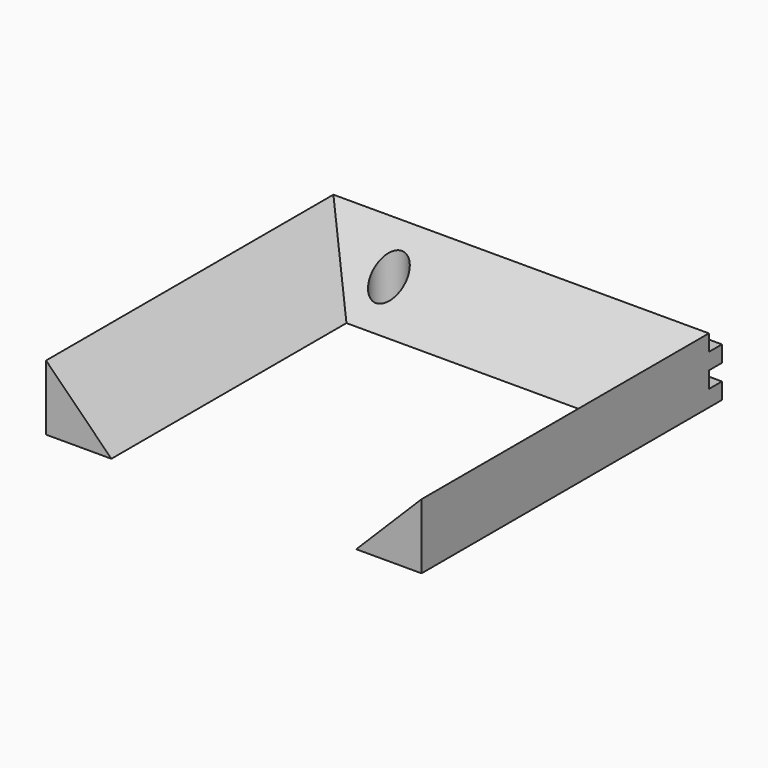
from build123d import *

# Parameters (mm, degrees)
F0_W     = 50.8
F0_H     = 228.6
F1_DEPTH = 50.8
F2_SIZE  = 50.79999
F4_R     = 12.7
F5_DEPTH = 63.5
F3_W     = 292.1
F3_H     = 12.7
F6_DEPTH = 12.7


# Not quite as in the source:
# - a fillet or chamfer is up to 0.001 mm smaller than in the source, because OpenCascade refuses the exact size


with BuildPart() as f1:
    # F0 (on Top) → F1 (new body)
    with BuildSketch(Plane.XY):
        with Locations((25.4, -114.3)):
            Rectangle(F0_W, F0_H)
        Polygon((0, 50.8), (0, 0), (50.8, 0), (241.3, 0), (292.1, 0), (292.1, 50.8), align=None)
        with Locations((266.7, -114.3)):
            Rectangle(F0_W, F0_H)
    extrude(amount=F1_DEPTH)

    # F2 (size 50.8 in the source; OpenCascade refuses exactly that, so slightly less here)
    f2_edges = [f1.edges().sort_by_distance(p)[0] for p in [
        (50.8, -114.3, 50.8),
        (146.05, 0, 50.8),
        (241.3, -114.3, 50.8),
    ]]
    chamfer(f2_edges, length=F2_SIZE)

    # F4 (on face) → F5 (cut)
    with BuildSketch(Plane(origin=(0, 0, 0), x_dir=(1, 0, 0), z_dir=(0, 0, -1))):
        with Locations((63.5, -25.4)):
            Circle(F4_R)
    extrude(amount=-F5_DEPTH, mode=Mode.SUBTRACT)

    # F3 (on face) → F6 (join)
    with BuildSketch(Plane(origin=(0, 50.8, 0), x_dir=(-1, 0, 0), z_dir=(0, 1, 0))):
        with Locations((-146.05, 6.35)):
            Rectangle(F3_W, F3_H)
        with Locations((-146.05, 31.75)):
            Rectangle(F3_W, F3_H)
    extrude(amount=F6_DEPTH)


solid = f1.part
